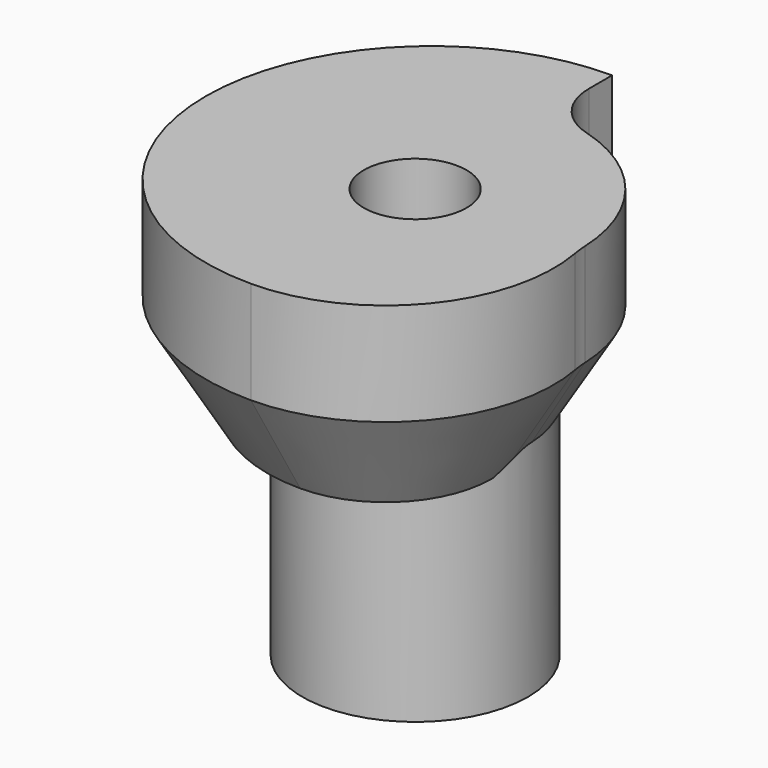
from build123d import *

# Parameters (mm, degrees)
F1_DEPTH      = 10
F2_R          = 5
F3_R          = 3
F4_T1_DEPTH   = 14.3477235542
F4_T4_ANGLE   = 100.2769257202
F4_T6_ANGLE   = 247.4672415992
F4_T8_ANGLE   = 7.8282705893
F4_T10_ANGLE  = 71.7247245492
F4_T12_ANGLE  = 74.1733798681
F5_R          = 5.5
F6_DEPTH      = 10
F6_DEPTH_BACK = 5
F7_R          = 2.5
F8_DEPTH      = 20.0010001


# Not quite as in the source:
# - a fillet or chamfer that OpenCascade refuses, or shapes differently, is made with other operations: its cross-section is extruded or revolved along the edge and cut away or added


with BuildPart() as f1:
    # F0 (on Top) → F1 (new body)
    with BuildSketch(Plane.XY):
        with BuildLine():
            ThreePointArc((0, 11.9994233124), (-8.123630239, 8.4157902443), (-10.9538720645, 0))
            ThreePointArc((-10.9538720645, 0), (-7.4157902443, -7.123630239), (0, -9.9994233124))
            ThreePointArc((0, -9.9994233124), (6.4028990813, -6.9221417854), (8, 0))
            ThreePointArc((8, 0), (5.6568542495, 5.6568542495), (0, 8))
            Line((0, 8), (0, 11.9994233124))
        make_face()
    extrude(amount=F1_DEPTH)

    # F2
    f2_edges = [f1.edges().sort_by_distance(p)[0] for p in [
        (8, 0, 5),
    ]]
    fillet(f2_edges, radius=F2_R)

    # F3
    f3_edges = [f1.edges().sort_by_distance(p)[0] for p in [
        (0, 8, 5),
    ]]
    fillet(f3_edges, radius=F3_R)

    # F4: chamfer of 5 x 3 on 5 edges, made by hand

    # F4_s2 → F4_t1 (cut)
    with BuildSketch(Plane.XZ.offset(-24.9307287984)):
        Polygon((0, 5), (-3, 0), (0, 0), align=None)
    extrude(amount=F4_T1_DEPTH, mode=Mode.SUBTRACT)

    # F4_s3 → F4_t4 (revolve, cut)
    with BuildSketch(Plane.YZ):
        Polygon((-9.9994233124, 5), (-6.9994233124, 0), (-9.9994233124, 0), align=None)
    revolve(axis=Axis((0, -1.7995271056, 0), (0, 0, 1)), revolution_arc=F4_T4_ANGLE, mode=Mode.SUBTRACT)

    # F4_s5 → F4_t6 (revolve, cut)
    with BuildSketch(Plane(origin=(-0.353957442, 0.8531488769, 0), x_dir=(0, 0, 1), z_dir=(0.3832115905, -0.9236605853, 0))):
        Polygon((5, -11.3826349029), (0, -8.3826349029), (0, -11.3826349029), align=None)
    revolve(axis=Axis((0, 1, 0), (0, 0, 1)), revolution_arc=F4_T6_ANGLE, mode=Mode.SUBTRACT)

    # F4_s7 → F4_t8 (revolve, cut)
    with BuildSketch(Plane(origin=(0.315895823, -1.7422505282, 0), x_dir=(0, 0, 1), z_dir=(0.1784059699, -0.9839569655, 0))):
        Polygon((5, -7.8788498285), (0, -4.8788498282), (0, -7.8788498282), align=None)
    revolve(axis=Axis((12.9881297006, 0.5554131457, 0), (0, 0, -1)), revolution_arc=F4_T8_ANGLE, mode=Mode.SUBTRACT)

    # F4_s9 → F4_t10 (revolve, cut)
    with BuildSketch(Plane(origin=(0, 0, 0), x_dir=(0, 0, 1), z_dir=(0.0427240892, -0.9990869092, 0))):
        Polygon((5, -8), (0, -5), (0, -8), align=None)
    revolve(axis=Axis((0, 0, 0), (0, 0, 1)), revolution_arc=F4_T10_ANGLE, mode=Mode.SUBTRACT)

    # F4_s11 → F4_t12 (revolve, cut)
    with BuildSketch(Plane(origin=(0, 0, 0), x_dir=(0, 0, 1), z_dir=(0.9620913858, -0.2727272727, 0))):
        Polygon((5, -8), (0, -5), (0, -8), align=None)
    revolve(axis=Axis((3, 10.5830052443, 0), (0, 0, -1)), revolution_arc=F4_T12_ANGLE, mode=Mode.SUBTRACT)

    # F5 (on face) → F6 (join, two sides)
    with BuildSketch(Plane.XY) as f6_sk:
        Circle(F5_R)
    extrude(amount=-F6_DEPTH)
    extrude(f6_sk.sketch, amount=F6_DEPTH_BACK)

    # F7 (on face) → F8 (cut, through all)
    with BuildSketch(Plane.XY.offset(10)):
        Circle(F7_R)
    extrude(amount=-F8_DEPTH, mode=Mode.SUBTRACT)


solid = f1.part
